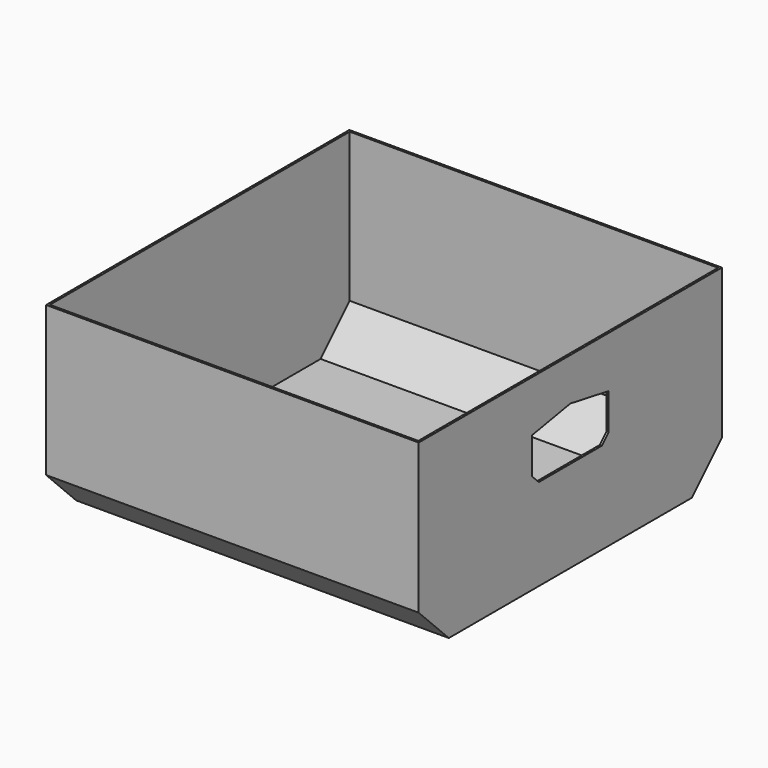
from build123d import *

# Parameters (mm, degrees)
F0_W        = 175
F0_H        = 178
F1_DEPTH    = 88
F2_SIZE     = 17.678
F3_T        = -1
F4_W        = 45
F4_H        = 25
F5_DEPTH    = 2
F6_T1_DEPTH = 1
F7_SIZE     = 4


# Not quite as in the source:
# - a fillet or chamfer that OpenCascade refuses, or shapes differently, is made with other operations: its cross-section is extruded or revolved along the edge and cut away or added


with BuildPart() as f1:
    # F0 (on Top) → F1 (new body)
    with BuildSketch(Plane.XY):
        with Locations((87.5, -89)):
            Rectangle(F0_W, F0_H)
    extrude(amount=F1_DEPTH)

    # F2
    f2_edges = [f1.edges().sort_by_distance(p)[0] for p in [
        (87.5, -178, 0),
        (87.5, 0, 0),
    ]]
    chamfer(f2_edges, length=F2_SIZE)

    # F3
    f3_openings = [f1.faces().sort_by_distance(p)[0] for p in [
        (87.5, -89, 88),
    ]]
    offset(amount=F3_T, openings=f3_openings)

    # F4 (on face) → F5 (cut)
    with BuildSketch(Plane.YZ.offset(175)):
        with Locations((-89, 55.5)):
            Rectangle(F4_W, F4_H)
    extrude(amount=-F5_DEPTH, mode=Mode.SUBTRACT)

    # F6: chamfer of 4 x 22.6851272785 on 2 edges, made by hand

    # F6_s2 → F6_t1 (join)
    with BuildSketch(Plane.YZ.offset(174)):
        Polygon((-111.5, 64), (-88.8148727215, 68), (-111.5, 68), align=None)
        Polygon((-66.5, 64), (-89.1851272785, 68), (-66.5, 68), align=None)
    extrude(amount=F6_T1_DEPTH)

    # F7
    f7_edges = [f1.edges().sort_by_distance(p)[0] for p in [
        (174.5, -111.5, 43),
        (174.5, -66.5, 43),
    ]]
    chamfer(f7_edges, length=F7_SIZE)


solid = f1.part
